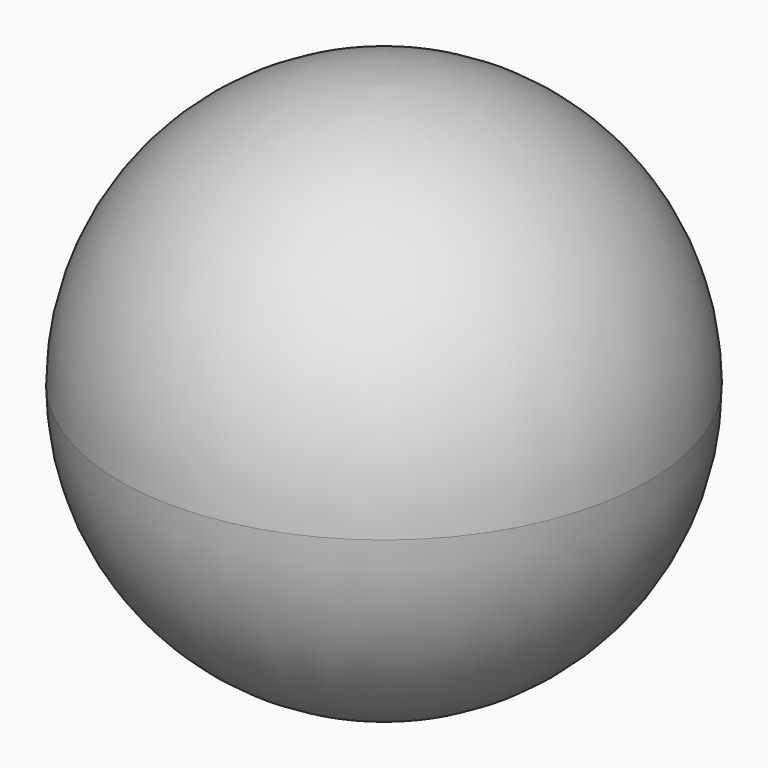
from build123d import *

# Parameters (mm, degrees)
F0_R     = 40
F1_DEPTH = 80
F2_R     = 39.99999


# Not quite as in the source:
# - a fillet or chamfer is up to 0.001 mm smaller than in the source, because OpenCascade refuses the exact size


with BuildPart() as f1:
    # F0 (on Top) → F1 (new body)
    with BuildSketch(Plane.XY):
        Circle(F0_R)
    extrude(amount=F1_DEPTH)

    # F2 (radius 40 in the source; OpenCascade refuses exactly that, so slightly less here)
    f2_edges = [f1.edges().sort_by_distance(p)[0] for p in [
        (-40, 0, 80),
        (-40, 0, 0),
    ]]
    fillet(f2_edges, radius=F2_R)


solid = f1.part
